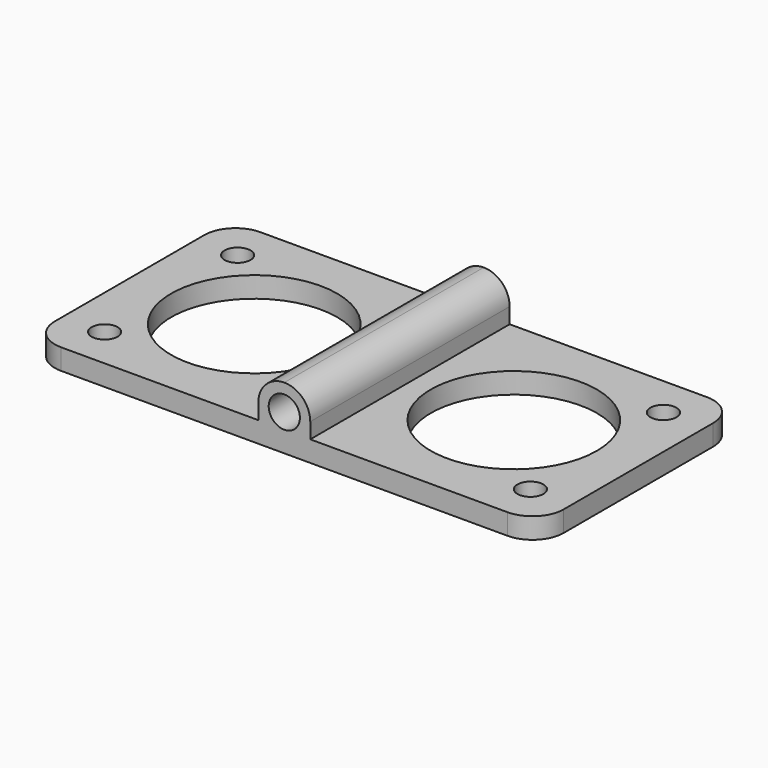
from build123d import *

# Parameters (mm, degrees)
F1_W      = 49
F1_H      = 24
F1_R      = 1.25
F2_DEPTH  = 2
F3_W      = 5
F3_H      = 24
F4_DEPTH  = 4
F5_R      = 1.5
F6_DEPTH  = 24
F7_R      = 2.49999
F8_R      = 3
F9_R      = 8
F10_DEPTH = 2


# Not quite as in the source:
# - a fillet or chamfer is up to 0.001 mm smaller than in the source, because OpenCascade refuses the exact size


with BuildPart() as f2:
    # F1 (on Top) → F2 (new body)
    with BuildSketch(Plane.XY):
        with Locations((-22.5, 10)):
            Rectangle(F1_W, F1_H)
        with Locations((-43, 2)):
            Circle(F1_R, mode=Mode.SUBTRACT)
        with Locations((-2, 2)):
            Circle(F1_R, mode=Mode.SUBTRACT)
        with Locations((-43, 18)):
            Circle(F1_R, mode=Mode.SUBTRACT)
        with Locations((-2, 18)):
            Circle(F1_R, mode=Mode.SUBTRACT)
    extrude(amount=F2_DEPTH)

    # F3 (on face) → F4 (join)
    with BuildSketch(Plane.XY.offset(2)):
        with Locations((-22.5, 10)):
            Rectangle(F3_W, F3_H)
    extrude(amount=F4_DEPTH)

    # F5 (on face) → F6 (cut, through all)
    with BuildSketch(Plane.XZ.offset(2)):
        with Locations((-22.5, 3.5)):
            Circle(F5_R)
    extrude(amount=-F6_DEPTH, mode=Mode.SUBTRACT)

    # F7 (radius 2.5 in the source; OpenCascade refuses exactly that, so slightly less here)
    f7_edges = [f2.edges().sort_by_distance(p)[0] for p in [
        (-20, 10, 6),
        (-25, 10, 6),
    ]]
    fillet(f7_edges, radius=F7_R)

    # F8
    f8_edges = [f2.edges().sort_by_distance(p)[0] for p in [
        (2, -2, 1),
        (2, 22, 1),
        (-47, 22, 1),
        (-47, -2, 1),
    ]]
    fillet(f8_edges, radius=F8_R)

    # F9 (on face) → F10 (cut, through all)
    with BuildSketch(Plane.XY.offset(2)):
        with Locations((-35, 10)):
            Circle(F9_R)
        with Locations((-10, 10)):
            Circle(F9_R)
    extrude(amount=-F10_DEPTH, mode=Mode.SUBTRACT)


solid = f2.part
